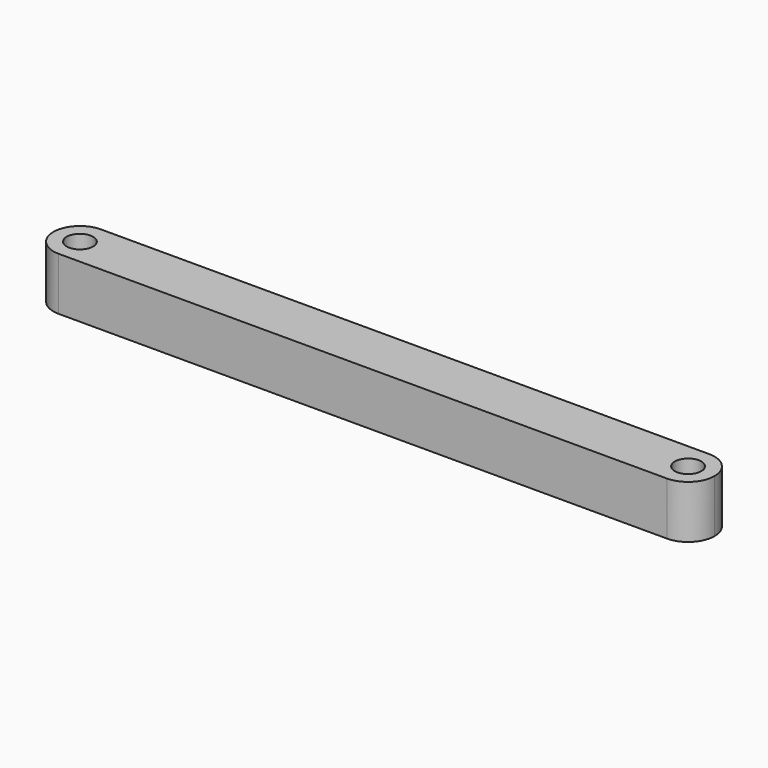
from build123d import *

# Parameters (mm, degrees)
F0_W     = 127
F0_H     = 10.16
F1_DEPTH = 10.16
F2_R     = 5.07999
F3_R     = 2.54
F4_DEPTH = 25.4


# Not quite as in the source:
# - a fillet or chamfer is up to 0.001 mm smaller than in the source, because OpenCascade refuses the exact size
# - a pattern or mirror of a feature is missing from the dataset's text; its kind, count and spacing are read off the source's solid


with BuildPart() as f1:
    # F0 (on Top) → F1 (new body)
    with BuildSketch(Plane.XY):
        Rectangle(F0_W, F0_H)
    extrude(amount=F1_DEPTH)

    # F2 (radius 5.08 in the source; OpenCascade refuses exactly that, so slightly less here)
    f2_edges = [f1.edges().sort_by_distance(p)[0] for p in [
        (-63.5, -5.08, 5.08),
        (-63.5, 5.08, 5.08),
        (63.5, -5.08, 5.08),
        (63.5, 5.08, 5.08),
    ]]
    fillet(f2_edges, radius=F2_R)

    # F3 (on face) → F4 (cut)
    with BuildSketch(Plane(origin=(0, 0, 0), x_dir=(1, 0, 0), z_dir=(0, 0, -1))):
        with Locations((-58.42, 0)):
            Circle(F3_R)
    f4 = extrude(amount=-F4_DEPTH, mode=Mode.SUBTRACT)

    # F4_copies: F4 across plane
    add(f4.mirror(Plane(origin=(0, 0, 0), x_dir=(0, 0, 1), z_dir=(1, 0, 0))), mode=Mode.SUBTRACT)


solid = f1.part
